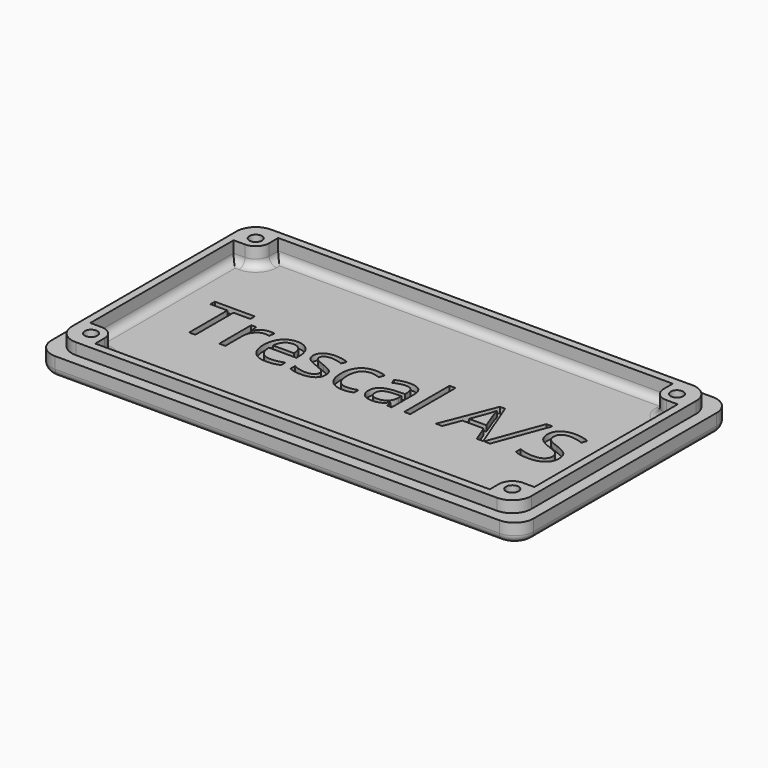
from build123d import *

# Parameters (mm, degrees)
F1_DEPTH       = 8
F2_DEPTH       = 5
F3_D           = 3.3
F3_CSINK_D     = 7.3
F3_CSINK_ANGLE = 90
F4_W           = 6.5
F4_H           = 47
F4_W_2         = 103.5
F4_H_2         = 6.5
F5_DEPTH       = 5
F6_R           = 3.5
F7_R           = 2
F8_TEXT_SIZE   = 19.5676766441
F9_DEPTH       = 1.5
F10_R          = 2


# Not quite as in the source:
# - Text() gives the source's letters only with a copy of the font that has no kerning and outlines rounded to 1/6400 em; it was checked with that copy


with BuildPart() as f1:
    # F0 (on Top) → F1 (new body)
    with BuildSketch(Plane.XY):
        with BuildLine():
            Line((-55.25, -32), (55.25, -32))
            ThreePointArc((55.25, -32), (58.7855339059, -30.5355339059), (60.25, -27))
            Line((60.25, -27), (60.25, 27))
            ThreePointArc((60.25, 27), (58.7855339059, 30.5355339059), (55.25, 32))
            Line((55.25, 32), (-55.25, 32))
            ThreePointArc((-55.25, 32), (-58.7855339059, 30.5355339059), (-60.25, 27))
            Line((-60.25, 27), (-60.25, -27))
            ThreePointArc((-60.25, -27), (-58.7855339059, -30.5355339059), (-55.25, -32))
        make_face()
    extrude(amount=F1_DEPTH)

    # F0 (on Top) → F2 (join)
    with BuildSketch(Plane.XY):
        with BuildLine():
            Line((-58.25, -35), (58.25, -35))
            ThreePointArc((58.25, -35), (61.7855339059, -33.5355339059), (63.25, -30))
            Line((63.25, -30), (63.25, 30))
            ThreePointArc((63.25, 30), (61.7855339059, 33.5355339059), (58.25, 35))
            Line((58.25, 35), (-58.25, 35))
            ThreePointArc((-58.25, 35), (-61.7855339059, 33.5355339059), (-63.25, 30))
            Line((-63.25, 30), (-63.25, -30))
            ThreePointArc((-63.25, -30), (-61.7855339059, -33.5355339059), (-58.25, -35))
        make_face()
        with BuildLine():
            ThreePointArc((60.25, -27), (58.7855339059, -30.5355339059), (55.25, -32))
            Line((55.25, -32), (-55.25, -32))
            ThreePointArc((-55.25, -32), (-58.7855339059, -30.5355339059), (-60.25, -27))
            Line((-60.25, -27), (-60.25, 27))
            ThreePointArc((-60.25, 27), (-58.7855339059, 30.5355339059), (-55.25, 32))
            Line((-55.25, 32), (55.25, 32))
            ThreePointArc((55.25, 32), (58.7855339059, 30.5355339059), (60.25, 27))
            Line((60.25, 27), (60.25, -27))
        make_face(mode=Mode.SUBTRACT)
    extrude(amount=F2_DEPTH)

    # F3 (through all)
    with Locations(Plane(origin=(0, 0, 0), x_dir=(1, 0, 0), z_dir=(0, 0, -1))):
        with Locations((-55.25, 27), (55.25, 27), (55.25, -27), (-55.25, -27)):
            CounterSinkHole(F3_D / 2, F3_CSINK_D / 2, counter_sink_angle=F3_CSINK_ANGLE)

    # F4 (on face) → F5 (cut)
    with BuildSketch(Plane.XY.offset(8)):
        with Locations((55, 0)):
            Rectangle(F4_W, F4_H)
        Rectangle(F4_W_2, F4_H)
        with Locations((0, 26.75)):
            Rectangle(F4_W_2, F4_H_2)
        with Locations((-55, 0)):
            Rectangle(F4_W, F4_H)
        with Locations((0, -26.75)):
            Rectangle(F4_W_2, F4_H_2)
    extrude(amount=-F5_DEPTH, mode=Mode.SUBTRACT)

    # F6
    f6_edges = [f1.edges().sort_by_distance(p)[0] for p in [
        (51.75, 23.5, 5.5),
        (51.75, -23.5, 5.5),
        (-51.75, -23.5, 5.5),
        (-51.75, 23.5, 5.5),
    ]]
    fillet(f6_edges, radius=F6_R)

    # F7
    f7_edges = [f1.edges().sort_by_distance(p)[0] for p in [
        (-61.785534, -33.535534, 0),
    ]]
    fillet(f7_edges, radius=F7_R)

    # F8 (on face) → F9 (cut)
    with BuildSketch(Plane.XY.offset(3)):
        with Locations((-50.396934445, -6.6489582408)):
            Text('Trescal A/S', F8_TEXT_SIZE, font='Open Sans', text_align=(TextAlign.LEFT, TextAlign.BOTTOM))
    extrude(amount=-F9_DEPTH, mode=Mode.SUBTRACT)

    # F10
    f10_edges = [f1.edges().sort_by_distance(p)[0] for p in [
        (0, 30, 3),
        (-52.775126, 24.525126, 3),
        (-58.25, 0, 3),
        (52.775126, 24.525126, 3),
        (-52.775126, -24.525126, 3),
        (0, -30, 3),
        (52.775126, -24.525126, 3),
        (58.25, 0, 3),
    ]]
    fillet(f10_edges, radius=F10_R)


solid = f1.part
